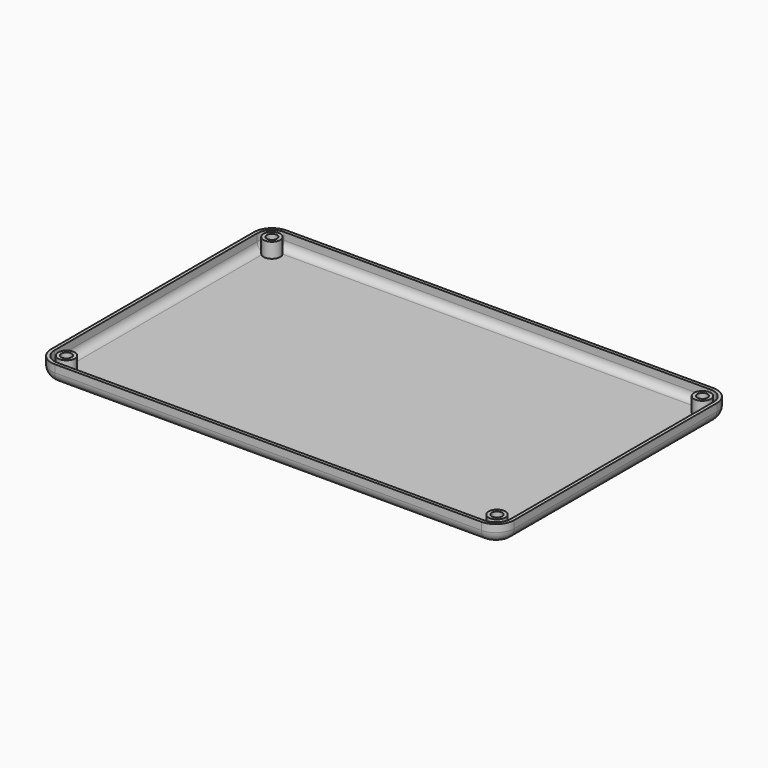
from build123d import *

# Parameters (mm, degrees)
F0_R         = 1.4
F1_DEPTH     = 5
F2_T1_DEPTH  = 69.5
F2_T3_DEPTH  = 117
F2_T6_ANGLE  = 90
F2_T8_ANGLE  = 90
F2_T10_ANGLE = 90
F2_T12_ANGLE = 90
F3_T         = 0.9


# Not quite as in the source:
# - a fillet or chamfer that OpenCascade refuses, or shapes differently, is made with other operations: its cross-section is extruded or revolved along the edge and cut away or added
# - a shell that OpenCascade refuses in one call is made with other operations: the cavity is built on its own and cut out


with BuildPart() as f1:
    # F0 (on Top) → F1 (new body)
    with BuildSketch(Plane.XY):
        with BuildLine():
            Line((82.8025215566, 53.4855341613), (-34.1974784434, 53.4855341613))
            ThreePointArc((-34.1974784434, 53.4855341613), (-37.7330123493, 52.0210680673), (-39.1974784434, 48.4855341613))
            Line((-39.1974784434, 48.4855341613), (-39.1974784434, -21.0144658387))
            ThreePointArc((-39.1974784434, -21.0144658387), (-37.7330123493, -24.5499997446), (-34.1974784434, -26.0144658387))
            Line((-34.1974784434, -26.0144658387), (82.8025215566, -26.0144658387))
            ThreePointArc((82.8025215566, -26.0144658387), (86.3380554625, -24.5499997446), (87.8025215566, -21.0144658387))
            Line((87.8025215566, -21.0144658387), (87.8025215566, 48.4855341613))
            ThreePointArc((87.8025215566, 48.4855341613), (86.3380554625, 52.0210680673), (82.8025215566, 53.4855341613))
        make_face()
        with Locations((-34.7974784434, -21.2644658387)):
            Circle(F0_R, mode=Mode.SUBTRACT)
        with Locations((83.3025215566, -21.2644658387)):
            Circle(F0_R, mode=Mode.SUBTRACT)
        with Locations((-34.7974784434, 49.1855341613)):
            Circle(F0_R, mode=Mode.SUBTRACT)
        with Locations((83.3025215566, 49.1855341613)):
            Circle(F0_R, mode=Mode.SUBTRACT)
    extrude(amount=F1_DEPTH)

    # F2: fillet of radius 3 on 8 edges, made by hand

    # F2_s2 → F2_t1 (cut)
    with BuildSketch(Plane.XZ.offset(-48.4855341613)):
        with BuildLine():
            ThreePointArc((87.8029215566, 3.0009656854), (86.9238419002, 0.8786796564), (84.8015558712, -0.0004))
            Line((84.8015558712, -0.0004), (84.8015558712, -0.3005365685))
            ThreePointArc((84.8015558712, -0.3005365685), (86.3020387139, -0.3001365685), (87.8025215566, -0.3001365685))
            Line((87.8025215566, -0.3001365685), (88.1026581252, 0))
            ThreePointArc((88.1026581252, 0), (88.1026581252, 1.5004828427), (88.1030581252, 3.0009656854))
            Line((88.1030581252, 3.0009656854), (87.8029215566, 3.0009656854))
        make_face()
        with BuildLine():
            ThreePointArc((-39.1978784434, 3.0009656854), (-38.3187987869, 0.8786796564), (-36.196512758, -0.0004))
            Line((-36.196512758, -0.0004), (-36.196512758, -0.3005365685))
            ThreePointArc((-36.196512758, -0.3005365685), (-37.6969956007, -0.3001365685), (-39.1974784434, -0.3001365685))
            Line((-39.1974784434, -0.3001365685), (-39.4976150119, 0))
            ThreePointArc((-39.4976150119, 0), (-39.4976150119, 1.5004828427), (-39.4980150119, 3.0009656854))
            Line((-39.4980150119, 3.0009656854), (-39.1978784434, 3.0009656854))
        make_face()
    extrude(amount=F2_T1_DEPTH, mode=Mode.SUBTRACT)

    # F2_s4 → F2_t3 (cut)
    with BuildSketch(Plane.YZ.offset(-34.1974784434)):
        with BuildLine():
            ThreePointArc((53.4859341613, 3.0009656854), (52.6068545049, 0.8786796564), (50.4845684759, -0.0004))
            Line((50.4845684759, -0.0004), (50.4845684759, -0.3005365685))
            ThreePointArc((50.4845684759, -0.3005365685), (51.9850513186, -0.3001365685), (53.4855341613, -0.3001365685))
            Line((53.4855341613, -0.3001365685), (53.7856707299, 0))
            ThreePointArc((53.7856707299, 0), (53.7856707299, 1.5004828427), (53.7860707299, 3.0009656854))
            Line((53.7860707299, 3.0009656854), (53.4859341613, 3.0009656854))
        make_face()
        with BuildLine():
            ThreePointArc((-26.0148658387, 3.0009656854), (-25.1357861822, 0.8786796564), (-23.0135001532, -0.0004))
            Line((-23.0135001532, -0.0004), (-23.0135001532, -0.3005365685))
            ThreePointArc((-23.0135001532, -0.3005365685), (-24.513982996, -0.3001365685), (-26.0144658387, -0.3001365685))
            Line((-26.0144658387, -0.3001365685), (-26.3146024072, 0))
            ThreePointArc((-26.3146024072, 0), (-26.3146024072, 1.5004828427), (-26.3150024072, 3.0009656854))
            Line((-26.3150024072, 3.0009656854), (-26.0148658387, 3.0009656854))
        make_face()
    extrude(amount=F2_T3_DEPTH, mode=Mode.SUBTRACT)

    # F2_s5 → F2_t6 (revolve, cut)
    with BuildSketch(Plane.XZ.offset(21.0144658387)):
        with BuildLine():
            ThreePointArc((-39.1978784434, 3.0009656854), (-38.3187987869, 0.8786796564), (-36.196512758, -0.0004))
            Line((-36.196512758, -0.0004), (-36.196512758, -0.3005365685))
            ThreePointArc((-36.196512758, -0.3005365685), (-37.6969956007, -0.3001365685), (-39.1974784434, -0.3001365685))
            Line((-39.1974784434, -0.3001365685), (-39.4976150119, 0))
            ThreePointArc((-39.4976150119, 0), (-39.4976150119, 1.5004828427), (-39.4980150119, 3.0009656854))
            Line((-39.4980150119, 3.0009656854), (-39.1978784434, 3.0009656854))
        make_face()
    revolve(axis=Axis((-34.1974784434, -21.0144658387, 0), (0, 0, 1)), revolution_arc=F2_T6_ANGLE, mode=Mode.SUBTRACT)

    # F2_s7 → F2_t8 (revolve, cut)
    with BuildSketch(Plane.XZ.offset(-48.4855341613)):
        with BuildLine():
            ThreePointArc((87.8029215566, 3.0009656854), (86.9238419002, 0.8786796564), (84.8015558712, -0.0004))
            Line((84.8015558712, -0.0004), (84.8015558712, -0.3005365685))
            ThreePointArc((84.8015558712, -0.3005365685), (86.3020387139, -0.3001365685), (87.8025215566, -0.3001365685))
            Line((87.8025215566, -0.3001365685), (88.1026581252, 0))
            ThreePointArc((88.1026581252, 0), (88.1026581252, 1.5004828427), (88.1030581252, 3.0009656854))
            Line((88.1030581252, 3.0009656854), (87.8029215566, 3.0009656854))
        make_face()
    revolve(axis=Axis((82.8025215566, 48.4855341613, 0), (0, 0, 1)), revolution_arc=F2_T8_ANGLE, mode=Mode.SUBTRACT)

    # F2_s9 → F2_t10 (revolve, cut)
    with BuildSketch(Plane.YZ.offset(-34.1974784434)):
        with BuildLine():
            ThreePointArc((53.4859341613, 3.0009656854), (52.6068545049, 0.8786796564), (50.4845684759, -0.0004))
            Line((50.4845684759, -0.0004), (50.4845684759, -0.3005365685))
            ThreePointArc((50.4845684759, -0.3005365685), (51.9850513186, -0.3001365685), (53.4855341613, -0.3001365685))
            Line((53.4855341613, -0.3001365685), (53.7856707299, 0))
            ThreePointArc((53.7856707299, 0), (53.7856707299, 1.5004828427), (53.7860707299, 3.0009656854))
            Line((53.7860707299, 3.0009656854), (53.4859341613, 3.0009656854))
        make_face()
    revolve(axis=Axis((-34.1974784434, 48.4855341613, 0), (0, 0, 1)), revolution_arc=F2_T10_ANGLE, mode=Mode.SUBTRACT)

    # F2_s11 → F2_t12 (revolve, cut)
    with BuildSketch(Plane.YZ.offset(82.8025215566)):
        with BuildLine():
            ThreePointArc((-26.0148658387, 3.0009656854), (-25.1357861822, 0.8786796564), (-23.0135001532, -0.0004))
            Line((-23.0135001532, -0.0004), (-23.0135001532, -0.3005365685))
            ThreePointArc((-23.0135001532, -0.3005365685), (-24.513982996, -0.3001365685), (-26.0144658387, -0.3001365685))
            Line((-26.0144658387, -0.3001365685), (-26.3146024072, 0))
            ThreePointArc((-26.3146024072, 0), (-26.3146024072, 1.5004828427), (-26.3150024072, 3.0009656854))
            Line((-26.3150024072, 3.0009656854), (-26.0148658387, 3.0009656854))
        make_face()
    revolve(axis=Axis((82.8025215566, -21.0144658387, 0), (0, 0, 1)), revolution_arc=F2_T12_ANGLE, mode=Mode.SUBTRACT)

    # F3: shell of thickness 0.9, made by hand


with BuildPart() as f3_core1:
    # F3_t2: copy of F1
    add(f1.part)

    # the walls: a layer under each face that stays
    f3_faces = [f3_core1.faces().sort_by_distance(p)[0] for p in [
        (86.3380554625, 52.0210680673, 3.9759831873),
        (85.7167351195, 51.3997477242, 0.878679657),
        (24.3025215566, 53.4855341613, 3.9759831877),
        (87.8025215566, 13.7355341613, 3.9759831873),
        (86.9238419005, 13.7355341613, 0.8786796567),
        (24.3025215566, 13.7355341614, 0),
        (81.9025215566, 49.1855341613, 2.5),
        (24.3025215566, 52.6068545055, 0.878679657),
        (-37.7330123493, 52.0210680673, 3.9759831864),
        (-39.1974784434, 13.7355341613, 3.9759831864),
        (-37.7330123493, -24.5499997446, 3.975983186),
        (24.3025215566, -26.0144658387, 3.975983186),
        (86.3380554625, -24.5499997446, 3.975983186),
        (-36.1974784434, -21.2644658387, 2.5),
        (81.9025215566, -21.2644658387, 2.5),
        (-36.1974784434, 49.1855341613, 2.5),
        (85.7167351192, -23.9286794012, 0.8786796567),
        (24.3025215566, -25.1357861816, 0.8786796558),
        (-37.1116920055, -23.9286794008, 0.8786796561),
        (-38.3187987866, 13.7355341613, 0.8786796561),
        (-37.1116920062, 51.3997477242, 0.878679657),
    ]]
    thicken(f3_faces, amount=-F3_T, mode=Mode.SUBTRACT)


with BuildPart() as f1_1:
    add(f1.part)

    # what is left inside the walls is the cavity
    f3_cavity = [f3_core1.part.solids().sort_by_distance(p)[0] for p in [
        (24.302522, 0.785534, 4.991),
    ]]
    add(f3_cavity, mode=Mode.SUBTRACT)


solid = f1_1.part
